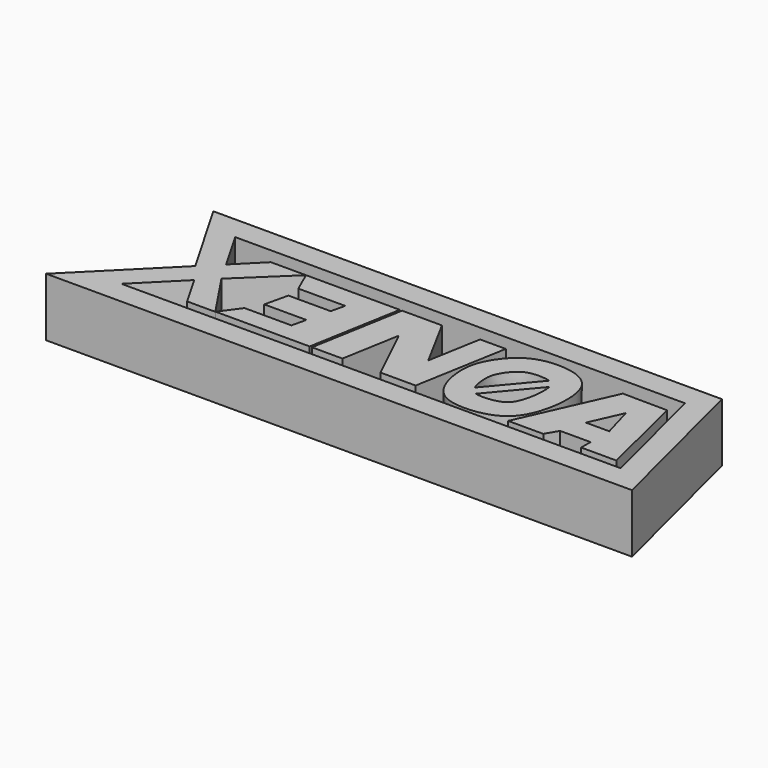
from build123d import *

# Parameters (mm, degrees)
F1_DEPTH = 25


# Not quite as in the source:
# - ends of sketch curves that miss each other by under 0.0002 mm in the source are joined
# - the dataset's text gives a spline's control points without its knots; the knots are read off the source's solid
# - a feature names something its author has since deleted; it is built from what else it names


with BuildPart() as f1:
    # F0 (on Top) → F1 (new body)
    with BuildSketch(Plane.XY):
        Polygon((35.3553390593, 35.3553390593), (0, 0), (250, 0), (232.3553390593, 69.9963552107), (15.3553390593, 69.9963552107), align=None)
        Polygon((32.6758509431, 59.9963530121), (224.56330661, 59.9963530121), (237.166372237, 10.0000021986), (24.1421409317, 10.0000021986), (41.4001874912, 27.2580487582), (47.8522307846, 33.7100920516), (42.6758487445, 42.6758487445), align=None, mode=Mode.SUBTRACT)
        Polygon((53.2824504623, 53.2824504623), (42.6758487445, 42.6758487445), (47.8522307846, 33.7100920516), (68.2824504623, 53.2824504623), align=None)
        Polygon((47.8522307846, 33.7100920516), (41.4001874912, 27.2580487582), (49.1933937334, 13.7598195929), (61.1933937334, 13.7598195929), align=None)
    extrude(amount=F1_DEPTH)


with BuildPart() as f1b:
    # F0 (on Top) → F1, piece 2 (new body)
    with BuildSketch(Plane.XY):
        Polygon((88.5540837341, 28.1308456181), (90.9036234209, 38.1308456181), (72.9036234209, 38.1308456181), (70.5540837341, 28.1308456181), align=None)
        Polygon((108.2824504623, 53.2824504623), (68.2824504623, 53.2824504623), (72.313347233, 44.1308456181), (92.313347233, 44.1308456181), (90.9036234209, 38.1308456181), (88.5540837341, 28.1308456181), (87.1034676285, 21.9568017674), (67.1034676285, 21.9568017674), (61.1933937334, 13.8901403418), (101.3365233556, 13.8901403418), align=None)
    extrude(amount=F1_DEPTH)


with BuildPart() as f1c:
    # F0 (on Top) → F1, piece 3 (new body)
    with BuildSketch(Plane.XY):
        Polygon((126.2824504623, 53.2824504623), (109.2824504623, 53.2824504623), (102.3365233556, 13.8901403418), (115.3365233556, 13.8901403418), (119.6777277973, 38.5103341671), (131.5355133201, 13.9200327762), (146.5355133201, 13.9200327762), (153.4814404268, 53.3123428967), (142.5191015005, 53.3123428967), (138.5251934142, 30.6617645774), align=None)
    extrude(amount=F1_DEPTH)


with BuildPart() as f1d:
    # F0 (on Top) → F1, piece 4 (new body)
    with BuildSketch(Plane.XY):
        with BuildLine():
            add(Edge.make_bspline(
                [(151.5315026045, 33.6161878365), (151.6881953051, 36.8603511522), (153.3257449913, 42.6794005447), (161.5552143615, 53.4867465492), (176.1548241084, 56.3217499328), (194.0088877696, 50.9134823684), (191.9976885112, 23.1984608195), (181.36266293, 11.4878216907), (160.3055787763, 10.4275817806), (152.5823075504, 20.9096175793), (151.3494491195, 29.8469552222), (151.5315026045, 33.6161878365)],
                knots=[0, 0, 0, 0, 0.0883183193, 0.1917010674, 0.3023367007, 0.4162516271, 0.5584218951, 0.6722296295, 0.7975352428, 0.8973873208, 1, 1, 1, 1], degree=3))
        make_face()
        with BuildLine():
            add(Edge.make_bspline(
                [(162.8184250503, 25.0692523461), (162.7388528349, 25.2709199434), (162.5250729743, 25.8491123795), (162.2111113791, 26.8772771924), (161.811446171, 28.5859325459), (161.5680124914, 30.3698864013), (161.490617043, 32.0313577817), (161.5032118997, 32.7877081125), (161.5198585813, 33.1337514359)],
                knots=[0.8971962129, 0.8971962129, 0.8971962129, 0.8971962129, 0.90625, 0.921875, 0.9375, 0.96875, 0.984375, 1, 1, 1, 1], degree=3))
            add(Edge.make_bspline(
                [(161.5198585813, 33.1337514359), (161.5365052629, 33.4797947593), (161.5904971328, 34.1076177221), (161.7198338174, 34.8971109654), (161.8983772283, 35.617959176), (162.1037900469, 36.2305480911), (162.3191108206, 36.7643620724), (162.5109148317, 37.1933987719), (162.7379267984, 37.6574642255), (163.0921353714, 38.326605495), (163.596210236, 39.1811127594), (164.287470415, 40.1970519056), (165.0414513207, 41.1551577869), (165.8327231283, 42.017135319), (166.4983498938, 42.6285934344), (167.0176778213, 43.0428000772), (167.3981141086, 43.3156806379), (167.7595288983, 43.5467960735), (168.1488651256, 43.766963423), (168.5654607343, 43.9738592368), (169.1603655772, 44.23185257), (169.9804869671, 44.5178805652), (171.0896341478, 44.7915612101), (172.3184150489, 44.9834054828), (173.6559028444, 45.0826399089), (174.7295299917, 45.0813201083), (175.4692709806, 45.0471315589), (175.9685909899, 45.0153875781), (176.5764482855, 44.960404607), (177.2752413398, 44.8700053931), (178.152789541, 44.7188709988), (178.7412145092, 44.5732668808), (179.0910574906, 44.4674492213), (179.0945257888, 44.4663980322)],
                knots=[0, 0, 0, 0, 0.015625, 0.03125, 0.046875, 0.0625, 0.0703125, 0.078125, 0.0859375, 0.09375, 0.109375, 0.125, 0.140625, 0.15625, 0.171875, 0.1796875, 0.1875, 0.1953125, 0.203125, 0.2109375, 0.21875, 0.234375, 0.25, 0.265625, 0.28125, 0.296875, 0.30078125, 0.3046875, 0.3125, 0.3203125, 0.328125, 0.34375, 0.3439066519, 0.3439066519, 0.3439066519, 0.3439066519], degree=3))
            add(Edge.make_bspline(
                [(179.0945257888, 44.4663980322), (179.4369974189, 44.3626000224), (180.0408289592, 44.137858269), (180.6603332198, 43.8043498556), (180.954614815, 43.5775919437), (181.1038370269, 43.4315691806), (181.1895827034, 43.3310307887), (181.2538264485, 43.2395291398), (181.3046724038, 43.1550069204), (181.3582155541, 43.05569095), (181.422796919, 42.9212624239), (181.5199173994, 42.6948431225), (181.7085595453, 42.1772024114), (181.8753089955, 41.5231873988), (181.9696544415, 41.0096622148), (181.9730783847, 40.9907957298)],
                knots=[0.3439066519, 0.3439066519, 0.3439066519, 0.3439066519, 0.359375, 0.375, 0.390625, 0.3984375, 0.40625, 0.4140625, 0.41796875, 0.421875, 0.42578125, 0.4296875, 0.4375, 0.453125, 0.4537178211, 0.4537178211, 0.4537178211, 0.4537178211], degree=3))
            add(Edge.make_bspline(
                [(181.9730783847, 40.9907957298), (182.0598994005, 40.512397778), (182.2045363428, 39.41183358), (182.2797979507, 37.4823107399), (182.193566141, 35.3678582229), (181.9493626032, 33.2017921364), (181.5644163989, 31.0887847577), (181.0667847965, 29.1323622869), (180.5011449009, 27.4494312491), (179.9317447836, 26.1476864655), (179.3824865747, 25.1785905134), (178.8685398921, 24.4779841747), (178.3709172748, 23.9520794031), (177.8264944089, 23.5060953751), (177.1374617731, 23.0738355235), (176.2112022482, 22.6358864412), (174.9558716393, 22.2007569681), (173.4559950281, 21.8323747048), (171.8198374216, 21.5722282716), (170.1442177268, 21.4412866926), (168.5280439261, 21.4466193999), (167.3160139795, 21.558065936), (166.4822451641, 21.6958640201), (166.0986472535, 21.7808626756), (165.9163137021, 21.8272428827), (165.8971010414, 21.8322026836)],
                knots=[0.4537178211, 0.4537178211, 0.4537178211, 0.4537178211, 0.46875, 0.484375, 0.5, 0.515625, 0.53125, 0.546875, 0.5625, 0.578125, 0.59375, 0.609375, 0.625, 0.640625, 0.65625, 0.671875, 0.6875, 0.703125, 0.71875, 0.734375, 0.75, 0.765625, 0.7734375, 0.78125, 0.7821827292, 0.7821827292, 0.7821827292, 0.7821827292], degree=3))
            add(Edge.make_bspline(
                [(165.8971010414, 21.8322026836), (165.7553892759, 21.868785963), (165.5531970067, 21.9272567748), (165.3254056153, 22.0041417656), (165.1739060305, 22.0612615773), (165.0494707627, 22.1134592968), (164.8977695401, 22.1837784003), (164.7376634219, 22.2699020236), (164.5740601511, 22.3743238889), (164.3757102389, 22.5229923761), (164.1329229874, 22.7478764528), (163.795317607, 23.1578632169), (163.4078371213, 23.7696356085), (163.0732924198, 24.4470716455), (162.8761783378, 24.9228825776), (162.8184250503, 25.0692523461)],
                knots=[0.7821827292, 0.7821827292, 0.7821827292, 0.7821827292, 0.7890625, 0.79296875, 0.796875, 0.80078125, 0.8046875, 0.8125, 0.8203125, 0.828125, 0.84375, 0.859375, 0.875, 0.890625, 0.8971962129, 0.8971962129, 0.8971962129, 0.8971962129], degree=3))
        make_face(mode=Mode.SUBTRACT)
        with BuildLine():
            add(Edge.make_bspline(
                [(179.0945257888, 44.4663980322), (179.4369974189, 44.3626000224), (180.0408289592, 44.137858269), (180.6603332198, 43.8043498556), (180.954614815, 43.5775919437), (181.1038370269, 43.4315691806), (181.1895827034, 43.3310307887), (181.2538264485, 43.2395291398), (181.3046724038, 43.1550069204), (181.3582155541, 43.05569095), (181.422796919, 42.9212624239), (181.5199173994, 42.6948431225), (181.7085595453, 42.1772024114), (181.8753089955, 41.5231873988), (181.9696544415, 41.0096622148), (181.9730783847, 40.9907957298)],
                knots=[0.3439066519, 0.3439066519, 0.3439066519, 0.3439066519, 0.359375, 0.375, 0.390625, 0.3984375, 0.40625, 0.4140625, 0.41796875, 0.421875, 0.42578125, 0.4296875, 0.4375, 0.453125, 0.4537178211, 0.4537178211, 0.4537178211, 0.4537178211], degree=3))
            Line((179.0945257888, 44.4663980322), (162.8183697977, 25.0692305451))
            add(Edge.make_bspline(
                [(165.8971010414, 21.8322026836), (165.7553892759, 21.868785963), (165.5531970067, 21.9272567748), (165.3254056153, 22.0041417656), (165.1739060305, 22.0612615773), (165.0494707627, 22.1134592968), (164.8977695401, 22.1837784003), (164.7376634219, 22.2699020236), (164.5740601511, 22.3743238889), (164.3757102389, 22.5229923761), (164.1329229874, 22.7478764528), (163.795317607, 23.1578632169), (163.4078371213, 23.7696356085), (163.0732924198, 24.4470716455), (162.8761783378, 24.9228825776), (162.8183697977, 25.0692305451)],
                knots=[0.7821827292, 0.7821827292, 0.7821827292, 0.7821827292, 0.7890625, 0.79296875, 0.796875, 0.80078125, 0.8046875, 0.8125, 0.8203125, 0.828125, 0.84375, 0.859375, 0.875, 0.890625, 0.8971962129, 0.8971962129, 0.8971962129, 0.8971962129], degree=3))
            Line((165.8971010414, 21.8322026836), (181.9730783847, 40.9907957298))
        make_face()
    extrude(amount=F1_DEPTH)


with BuildPart() as f1e:
    # F0 (on Top) → F1, piece 5 (new body)
    with BuildSketch(Plane.XY):
        Polygon((232.5355133201, 13.4541621667), (223.0829559751, 52.321232543), (204.0839364723, 52.5142556785), (186.5355133201, 13.258009744), (201.5355133201, 13.258009744), (204.5355133201, 18.4541621667), (217.5355133201, 18.4541621667), (217.5355133201, 13.4541621667), align=None)
        Polygon((213.6570562804, 42.148201446), (217.5355133201, 28.4541621667), (207.5355133201, 28.4541621667), align=None, mode=Mode.SUBTRACT)
    extrude(amount=F1_DEPTH)


solid = Compound([f1.part, f1b.part, f1c.part, f1d.part, f1e.part])
